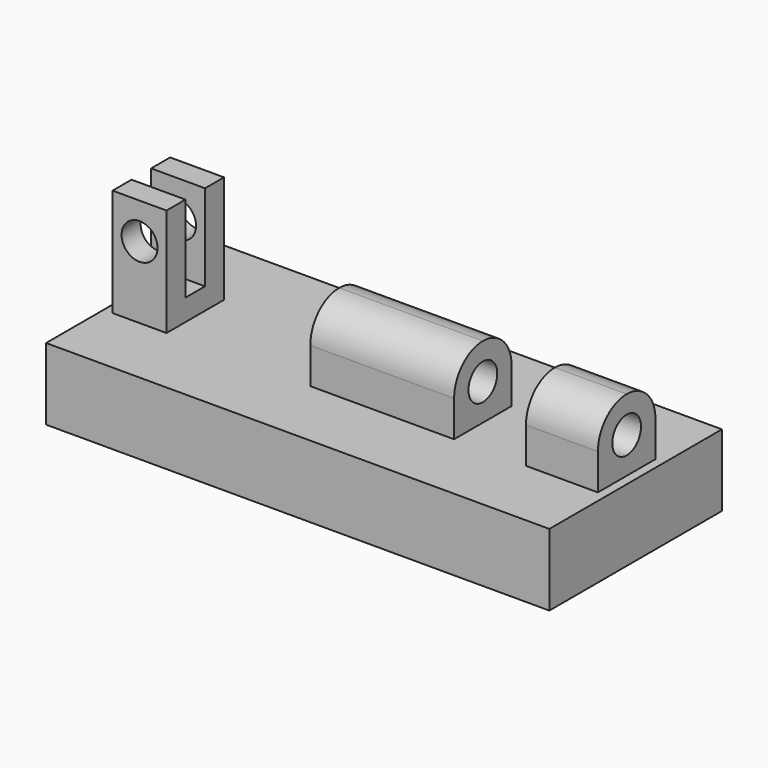
from build123d import *

# Parameters (mm, degrees)
F0_W      = 177.8
F0_H      = 76.2
F1_DEPTH  = 25.4
F2_W      = 19.05
F2_H      = 38.1
F2_W_2    = 50.8
F2_H_2    = 25.4
F2_W_3    = 25.4
F3_DEPTH  = 25.4
F4_R      = 6.35
F5_DEPTH  = 101.6
F6_R      = 12.69999
F7_W      = 8.636
F7_H      = 30.48
F8_DEPTH  = 25.4
F9_R      = 6.35
F10_DEPTH = 25.4


# Not quite as in the source:
# - a fillet or chamfer is up to 0.001 mm smaller than in the source, because OpenCascade refuses the exact size


with BuildPart() as f1:
    # F0 (on Top) → F1 (new body)
    with BuildSketch(Plane.XY):
        with Locations((0, -12.7)):
            Rectangle(F0_W, F0_H)
    extrude(amount=F1_DEPTH)

    # F2 (on Front) → F3 (join)
    with BuildSketch(Plane.XZ):
        with Locations((-76.2, 44.45)):
            Rectangle(F2_W, F2_H)
        with Locations((9.525, 38.1)):
            Rectangle(F2_W_2, F2_H_2)
        with Locations((73.025, 38.1)):
            Rectangle(F2_W_3, F2_H_2)
    extrude(amount=F3_DEPTH)

    # F4 (on face) → F5 (cut, through all)
    with BuildSketch(Plane.YZ.offset(85.725)):
        with Locations((-12.7, 38.1)):
            Circle(F4_R)
    extrude(amount=-F5_DEPTH, mode=Mode.SUBTRACT)

    # F6 (radius 12.7 in the source; OpenCascade refuses exactly that, so slightly less here)
    f6_edges = [f1.edges().sort_by_distance(p)[0] for p in [
        (9.525, -25.4, 50.8),
        (9.525, 0, 50.8),
        (73.025, -25.4, 50.8),
        (73.025, 0, 50.8),
    ]]
    fillet(f6_edges, radius=F6_R)

    # F7 (on face) → F8 (cut)
    with BuildSketch(Plane(origin=(-85.725, 0, 0), x_dir=(0, -1, 0), z_dir=(-1, 0, 0))):
        with Locations((12.7, 48.26)):
            Rectangle(F7_W, F7_H)
    extrude(amount=-F8_DEPTH, mode=Mode.SUBTRACT)

    # F9 (on face) → F10 (cut)
    with BuildSketch(Plane.XZ.offset(25.4)):
        with Locations((-76.2, 50.8)):
            Circle(F9_R)
    extrude(amount=-F10_DEPTH, mode=Mode.SUBTRACT)


solid = f1.part
